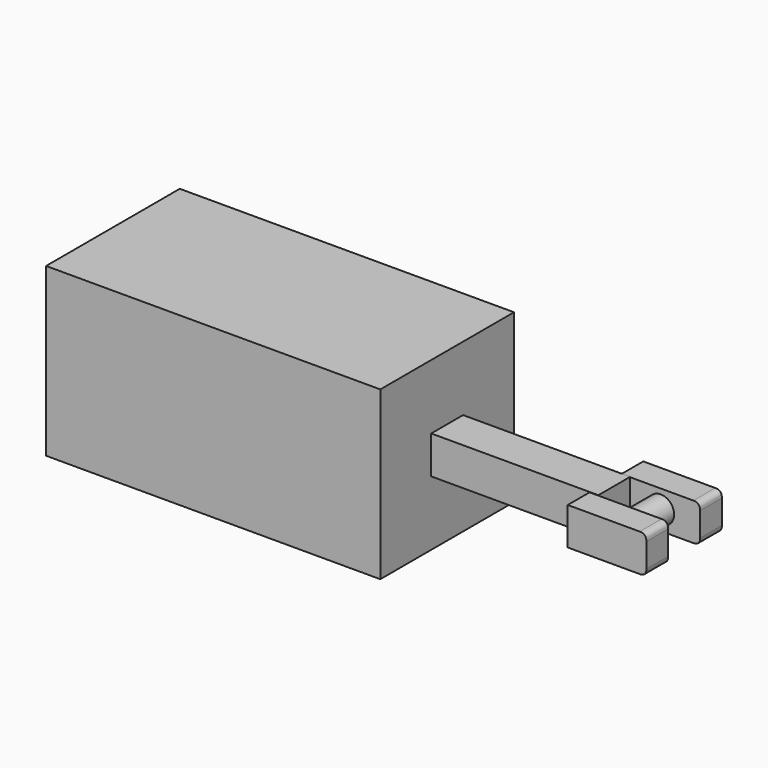
from build123d import *

# Parameters (mm, degrees)
F0_W         = 12.7
F0_H         = 12.7
F1_DEPTH     = 25.4
F2_R         = 5.5626
F3_DEPTH     = 19.05
F4_W         = 3.0250146519
F4_H         = 2.872077981
F5_DEPTH     = 12.7
F7_DEPTH     = 2.8448
F8_R         = 1.016
F9_DEPTH     = 5.2832
F10_T1_DEPTH = 4.6143001951
F10_T3_DEPTH = 4.6143001951


# Not quite as in the source:
# - a fillet or chamfer that OpenCascade refuses, or shapes differently, is made with other operations: its cross-section is extruded or revolved along the edge and cut away or added


with BuildPart() as f1:
    # F0 (on Right) → F1 (new body)
    with BuildSketch(Plane.YZ):
        Rectangle(F0_W, F0_H)
    extrude(amount=-F1_DEPTH)

    # F2 (on face) → F3 (cut)
    with BuildSketch(Plane(origin=(-25.4, 0, 0), x_dir=(0, -1, 0), z_dir=(-1, 0, 0))):
        Circle(F2_R)
    extrude(amount=-F3_DEPTH, mode=Mode.SUBTRACT)

    # F4 (on face) → F5 (join)
    with BuildSketch(Plane.YZ):
        Rectangle(F4_W, F4_H)
    extrude(amount=F5_DEPTH)

    # F6 (on face) → F7 (join)
    with BuildSketch(Plane(origin=(0, 0, -1.4360389905), x_dir=(1, 0, 0), z_dir=(0, 0, -1))):
        Polygon((12.0346518233, 3.5868075211), (12.0346518233, 1.512507326), (12.7, 1.512507326), (18.0126260966, 1.512507326), (18.0126260966, 3.5868075211), align=None)
        Polygon((18.0126260966, -1.512507326), (12.7, -1.512507326), (12.0346518233, -1.512507326), (12.0346518233, -3.5868075211), (18.0126260966, -3.5868075211), align=None)
    extrude(amount=-F7_DEPTH)

    # F8 (on face) → F9 (join)
    with BuildSketch(Plane.XZ.offset(3.5868075211)):
        with Locations((15.02363896, 0)):
            Circle(F8_R)
    extrude(amount=-F9_DEPTH)

    # F10: fillet of radius 0.508 on 4 edges, made by hand

    # F10_s2 → F10_t1 (cut)
    with BuildSketch(Plane.XZ.offset(0.242507326)):
        with BuildLine():
            add(Edge.make_bspline(
                [(17.5046260966, -1.4360389905), (18.0126260966, -1.4360389905), (18.0126260966, -0.9280389905)],
                knots=[0, 0, 0, 1, 1, 1], degree=2, weights=[1, 1, 1]))
            Line((18.0126260966, -0.9280389905), (18.0126260966, -1.4360389905))
            Line((18.0126260966, -1.4360389905), (17.5046260966, -1.4360389905))
        make_face()
        with BuildLine():
            add(Edge.make_bspline(
                [(18.0126260966, 0.9007610095), (18.0126260966, 1.4087610095), (17.5046260966, 1.4087610095)],
                knots=[0, 0, 0, 1, 1, 1], degree=2, weights=[1, 1, 1]))
            Line((17.5046260966, 1.4087610095), (18.0126260966, 1.4087610095))
            Line((18.0126260966, 1.4087610095), (18.0126260966, 0.9007610095))
        make_face()
    extrude(amount=F10_T1_DEPTH, mode=Mode.SUBTRACT)

    # F10_s4 → F10_t3 (cut)
    with BuildSketch(Plane.XZ.offset(-4.8568075211)):
        with BuildLine():
            add(Edge.make_bspline(
                [(17.5046260966, -1.4360389905), (18.0126260966, -1.4360389905), (18.0126260966, -0.9280389905)],
                knots=[0, 0, 0, 1, 1, 1], degree=2, weights=[1, 1, 1]))
            Line((18.0126260966, -0.9280389905), (18.0126260966, -1.4360389905))
            Line((18.0126260966, -1.4360389905), (17.5046260966, -1.4360389905))
        make_face()
        with BuildLine():
            add(Edge.make_bspline(
                [(18.0126260966, 0.9007610095), (18.0126260966, 1.4087610095), (17.5046260966, 1.4087610095)],
                knots=[0, 0, 0, 1, 1, 1], degree=2, weights=[1, 1, 1]))
            Line((17.5046260966, 1.4087610095), (18.0126260966, 1.4087610095))
            Line((18.0126260966, 1.4087610095), (18.0126260966, 0.9007610095))
        make_face()
    extrude(amount=F10_T3_DEPTH, mode=Mode.SUBTRACT)


solid = f1.part
